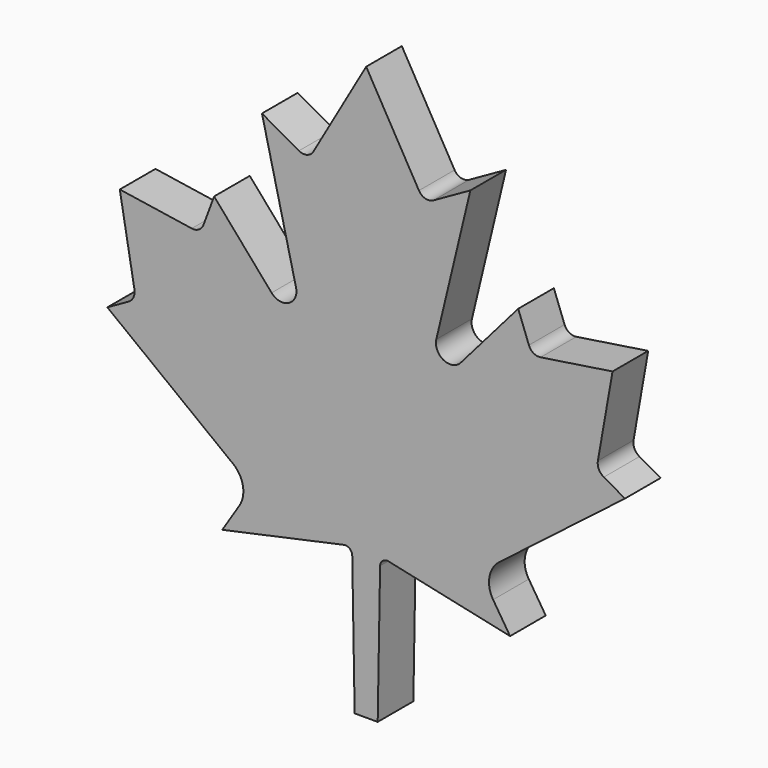
from build123d import *

# Parameters (mm, degrees)
F1_DEPTH = 1.6
F2_SCALE = 1.25


with BuildPart() as f1:
    # F0 (on Front) → F1 (new body)
    with BuildSketch(Plane.XZ):
        with BuildLine():
            Line((0, 0), (0.413425887, 0))
            Line((0.413425887, 0), (0.8268517741, 0))
            Line((0.8268517741, 0), (0.913425887, 4.9598276104))
            ThreePointArc((0.913425887, 4.9598276104), (1.0081087659, 5.1513941345), (1.2162387154, 5.1998142211))
            Line((1.2162387154, 5.1998142211), (5.5792679741, 4.2561256))
            Line((5.5792679741, 4.2561256), (4.9705727128, 5.2097686))
            ThreePointArc((4.9705727128, 5.2097686), (4.8360238518, 5.8823080691), (5.1909015741, 6.4692276))
            Line((5.1909015741, 6.4692276), (9.7032877741, 9.9448366))
            Line((9.7032877741, 9.9448366), (8.9429137741, 10.373741))
            ThreePointArc((8.9429137741, 10.373741), (8.7655752428, 10.5643141825), (8.7308237651, 10.8223053206))
            Line((8.7308237651, 10.8223053206), (9.2566129031, 13.8156465299))
            Line((9.2566129031, 13.8156465299), (6.6742096902, 13.4228908506))
            ThreePointArc((6.6742096902, 13.4228908506), (6.4203753707, 13.4717678019), (6.2541926873, 13.66976814))
            Line((6.2541926873, 13.66976814), (5.8709357741, 14.6970242))
            Line((5.8709357741, 14.6970242), (3.8084164021, 12.3209425283))
            ThreePointArc((3.8084164021, 12.3209425283), (3.1924630132, 12.2021834474), (2.9307614756, 12.7722839665))
            Line((2.9307614756, 12.7722839665), (4.1535767314, 17.8771898961))
            Line((4.1535767314, 17.8771898961), (2.8251496269, 17.1293843238))
            ThreePointArc((2.8251496269, 17.1293843238), (2.5371995805, 17.0940398171), (2.3078402562, 17.2716876815))
            Line((2.3078402562, 17.2716876815), (0.413425887, 20.5711957021))
            Line((0.413425887, 20.5711957021), (-1.4809884821, 17.2716876815))
            ThreePointArc((-1.4809884821, 17.2716876815), (-1.7103478064, 17.0940398171), (-1.9982978528, 17.1293843238))
            Line((-1.9982978528, 17.1293843238), (-3.3267249573, 17.8771898961))
            Line((-3.3267249573, 17.8771898961), (-2.1039097015, 12.7722839665))
            ThreePointArc((-2.1039097015, 12.7722839665), (-2.3656112391, 12.2021834474), (-2.9815646281, 12.3209425283))
            Line((-2.9815646281, 12.3209425283), (-5.044084, 14.6970242))
            Line((-5.044084, 14.6970242), (-5.4273409133, 13.66976814))
            ThreePointArc((-5.4273409133, 13.66976814), (-5.5935235967, 13.4717678019), (-5.8473579162, 13.4228908506))
            Line((-5.8473579162, 13.4228908506), (-8.4297611291, 13.8156465299))
            Line((-8.4297611291, 13.8156465299), (-7.903971991, 10.8223053206))
            ThreePointArc((-7.903971991, 10.8223053206), (-7.9387234687, 10.5643141825), (-8.116062, 10.373741))
            Line((-8.116062, 10.373741), (-8.876436, 9.9448366))
            Line((-8.876436, 9.9448366), (-4.3640498, 6.4692276))
            ThreePointArc((-4.3640498, 6.4692276), (-4.0091720777, 5.8823080691), (-4.1437209388, 5.2097686))
            Line((-4.1437209388, 5.2097686), (-4.7524162, 4.2561256))
            Line((-4.7524162, 4.2561256), (-0.3893869413, 5.1998142211))
            ThreePointArc((-0.3893869413, 5.1998142211), (-0.1812569918, 5.1513941345), (-0.086574113, 4.9598276104))
            Line((-0.086574113, 4.9598276104), (0, 0))
        make_face()
    extrude(amount=F1_DEPTH)


with BuildPart() as f1_1:
    # F2: moved
    add(f1.part.scale(F2_SCALE).moved(Location((-0.2067129435, 0.4, 0))))


solid = f1_1.part
